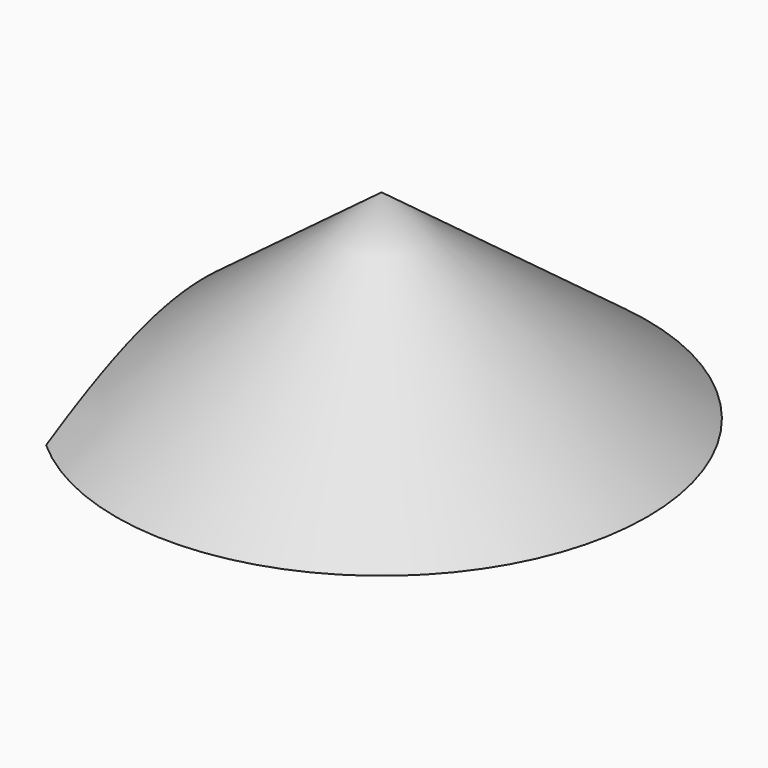
from build123d import *

# Parameters (mm, degrees)
F3_DEPTH       = 5
F3_DEPTH_BACK  = 50
F4_DEPTH       = 30
F7_DEPTH       = 5
F7_DEPTH_BACK  = 5
F10_DEPTH      = 5
F10_DEPTH_BACK = 5
F12_DEPTH      = 20


# Not quite as in the source:
# - a feature names something its author has since deleted; it is built from what else it names


with BuildPart() as f1:
    # F0 (on Front) → F1 (revolve)
    with BuildSketch(Plane.XZ):
        Polygon((0, 37.5), (0, 30), (10, 30), align=None)
    revolve(axis=Axis((0, 0, 33.75), (0, 0, 1)))

    # F2 (on Top) → F3 (cut, two sides)
    with BuildSketch(Plane.XY) as f3_sk:
        with BuildLine():
            Line((-6.644110661, 4.455984013), (-6.644110661, 7.4998452328))
            Line((-6.644110661, 7.4998452328), (-11.5474741906, 7.4998452328))
            Line((-11.5474741906, 7.4998452328), (-11.5474741906, -9.0728485957))
            Line((-11.5474741906, -9.0728485957), (-6.644110661, -9.0728485957))
            Line((-6.644110661, -9.0728485957), (-6.644110661, -4.455984013))
            ThreePointArc((-6.644110661, -4.455984013), (-8, 0), (-6.644110661, 4.455984013))
        make_face()
        with BuildLine():
            Line((-6.644110661, -4.455984013), (-6.644110661, 4.455984013))
            ThreePointArc((-6.644110661, 4.455984013), (-8, 0), (-6.644110661, -4.455984013))
        make_face()
    extrude(amount=-F3_DEPTH, mode=Mode.SUBTRACT)
    extrude(f3_sk.sketch, amount=F3_DEPTH_BACK, mode=Mode.SUBTRACT)

    # F2 (on Top) → F4 (cut)
    with BuildSketch(Plane.XY):
        with BuildLine():
            ThreePointArc((8, 0), (2.3288532277, 7.6535248509), (-6.644110661, 4.455984013))
            Line((-6.644110661, 4.455984013), (-6.644110661, -4.455984013))
            ThreePointArc((-6.644110661, -4.455984013), (2.3288532277, -7.6535248509), (8, 0))
        make_face()
    extrude(amount=F4_DEPTH, mode=Mode.SUBTRACT)

    # F6 (on line) → F7 (cut, two sides)
    with BuildSketch(Plane(origin=(3.1843009926, -8.1633897791, 0), x_dir=(-0.9316321862, -0.3634026275, 0), z_dir=(-0.3634026275, 0.9316321862, 0))) as f7_sk:
        with BuildLine():
            ThreePointArc((0, 28), (-4.026334039, 15), (0, 2))
            ThreePointArc((0, 2), (4.026334039, 15), (0, 28))
        make_face()
    extrude(amount=F7_DEPTH, mode=Mode.SUBTRACT)
    extrude(f7_sk.sketch, amount=-F7_DEPTH_BACK, mode=Mode.SUBTRACT)

    # F9 (on line) → F10 (cut, two sides)
    with BuildSketch(Plane(origin=(3.1843009926, 8.1633897791, 0), x_dir=(0.9316321862, -0.3634026275, 0), z_dir=(-0.3634026275, -0.9316321862, 0))) as f10_sk:
        with BuildLine():
            ThreePointArc((0, 28), (-4.026334039, 15), (0, 2))
            ThreePointArc((0, 2), (4.026334039, 15), (0, 28))
        make_face()
    extrude(amount=-F10_DEPTH, mode=Mode.SUBTRACT)
    extrude(f10_sk.sketch, amount=F10_DEPTH_BACK, mode=Mode.SUBTRACT)

    # F11 (on Right) → F12 (cut)
    with BuildSketch(Plane.YZ):
        with BuildLine():
            ThreePointArc((0, 28), (-4.026334039, 15), (0, 2))
            ThreePointArc((0, 2), (4.026334039, 15), (0, 28))
        make_face()
    extrude(amount=F12_DEPTH, mode=Mode.SUBTRACT)


solid = f1.part
